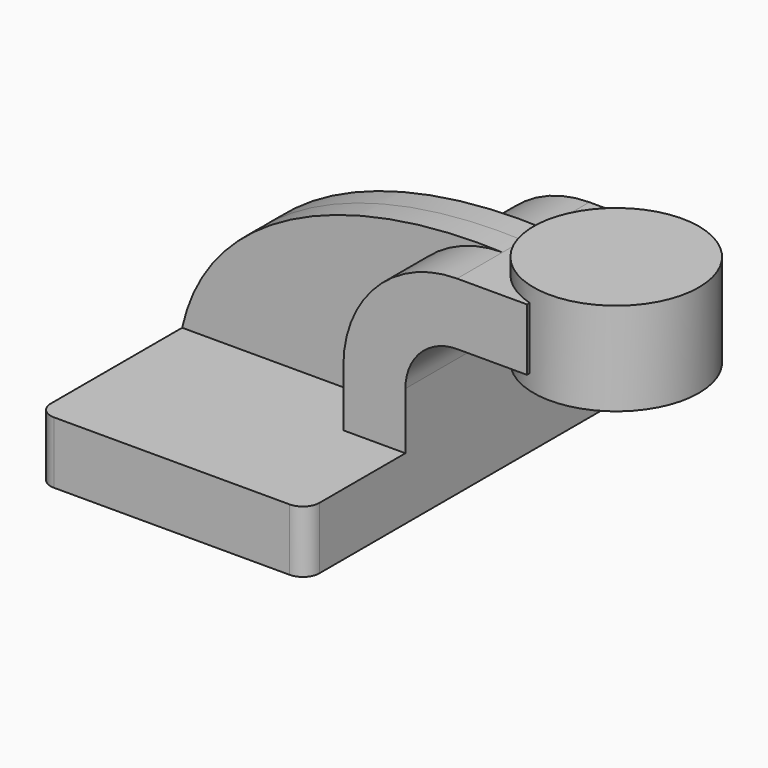
from build123d import *

# Parameters (mm, degrees)
F1_DEPTH = 63.5
F0_W     = 18.3103905071
F0_H     = 19.05
F2_DEPTH = 25.4
F3_DEPTH = 7.9375
F0_W_2   = 25.4
F0_H_2   = 28.575
F5_R     = 5.08


# Not quite as in the source:
# - a feature names something its author has since deleted; it is built from what else it names


with BuildPart() as f1:
    # F0 (on Front) → F1 (new body, symmetric)
    with BuildSketch(Plane.XZ):
        Polygon((-41.275, -9.525), (41.275, -9.525), (41.275, 9.525), (22.225, 9.525), (-41.275, 9.525), align=None)
    extrude(amount=F1_DEPTH, both=True)

    # F0 (on Front) → F2 (join, symmetric)
    with BuildSketch(Plane.XZ):
        with BuildLine():
            Line((22.225, 9.525), (41.275, 9.525))
            Line((41.275, 9.525), (41.275, 27.0002))
            ThreePointArc((41.275, 27.0002), (45.9246798487, 38.2255201513), (57.15, 42.8752))
            Line((57.15, 42.8752), (60.325, 42.8752))
            Line((60.325, 42.8752), (60.325, 61.9252))
            Line((60.325, 61.9252), (57.15, 61.9252))
            ThreePointArc((57.15, 61.9252), (32.4542956671, 51.6959043329), (22.225, 27.0002))
            Line((22.225, 27.0002), (22.225, 9.525))
        make_face()
        with Locations((69.4801952536, 52.4002)):
            Rectangle(F0_W, F0_H)
    extrude(amount=F2_DEPTH, both=True)

    # F0 (on Front) → F3 (join, symmetric)
    with BuildSketch(Plane.XZ):
        with BuildLine():
            add(Edge.make_bspline(
                [(-41.275, 9.525), (-33.2450978458, 46.1078099906), (9.6913008019, 63.8398453593), (57.15, 61.9252)],
                knots=[0, 0, 0, 0, 111.5045361635, 111.5045361635, 111.5045361635, 111.5045361635], degree=3))
            Line((-41.275, 9.525), (22.225, 9.525))
            Line((22.225, 9.525), (22.225, 27.0002))
            ThreePointArc((22.225, 27.0002), (32.4542956671, 51.6959043329), (57.15, 61.9252))
        make_face()
    extrude(amount=F3_DEPTH, both=True)

    # F0 (on Front) → F4 (revolve)
    with BuildSketch(Plane.XZ):
        with Locations((98.425, 52.4808056653)):
            Rectangle(F0_W_2, F0_H_2)
    revolve(axis=Axis((85.725, 0, 52.4808056653), (0, 0, 1)))

    # F5
    f5_edges = [f1.edges().sort_by_distance(p)[0] for p in [
        (41.275, -63.5, 0),
        (41.275, 63.5, 0),
        (-41.275, 63.5, 0),
        (-41.275, -63.5, 0),
    ]]
    fillet(f5_edges, radius=F5_R)


solid = f1.part
